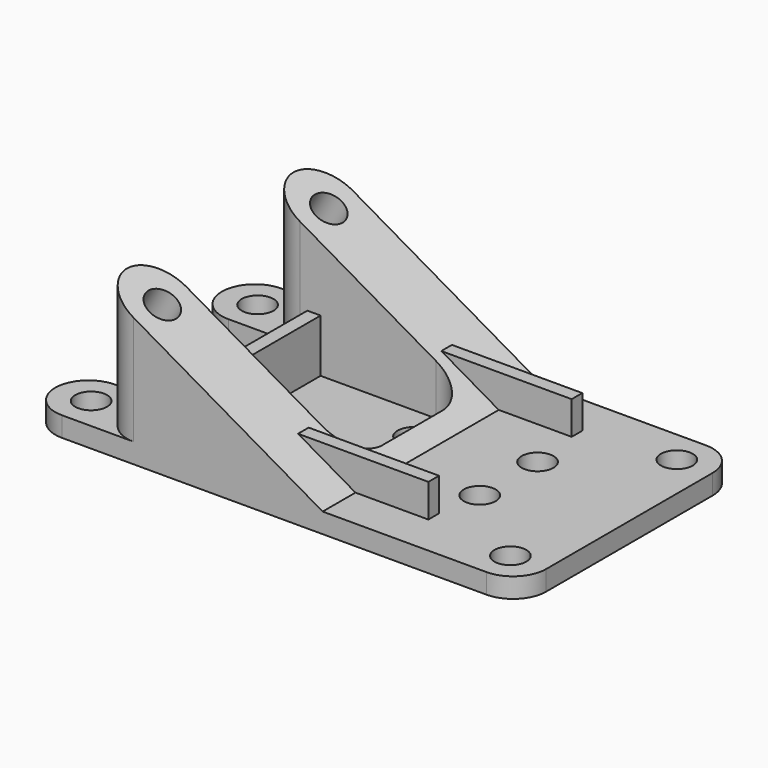
from build123d import *

# Parameters (mm, degrees)
F0_W        = 3
F0_H        = 5
F1_DEPTH    = 25
F0_R        = 2.4
F2_DEPTH    = 3
F3_T4_DEPTH = 238.5325445422
F4_R        = 4.99999
F5_R        = 4.99999
F6_R        = 5
F8_DEPTH    = 5
F9_ANGLE    = -30
F10_ANGLE   = -30
F7_W        = 36.4
F7_H        = 25
F7_R        = 4.4
F7_R_2      = 2.4
F13_DEPTH   = 2
F14_DEPTH   = 8


# Not quite as in the source:
# - a fillet or chamfer that OpenCascade refuses, or shapes differently, is made with other operations: its cross-section is extruded or revolved along the edge and cut away or added
# - a fillet or chamfer is up to 0.001 mm smaller than in the source, because OpenCascade refuses the exact size


with BuildPart() as f1:
    # F0 (on Top) → F1 (new body)
    with BuildSketch(Plane.XY):
        Polygon((-26.2931033156, 20.6850649182), (-26.2931033156, 15.6850649182), (-26.2931033156, 10.6850649182), (4.2068966844, 10.6850649182), (4.2068966844, 15.6850649182), (4.2068966844, 20.6850649182), align=None)
        with BuildLine():
            ThreePointArc((-18.8931033156, 15.6850649182), (-21.2931033156, 13.2850649182), (-23.6931033156, 15.6850649182))
            ThreePointArc((-23.6931033156, 15.6850649182), (-21.2931033156, 18.0850649182), (-18.8931033156, 15.6850649182))
        make_face(mode=Mode.SUBTRACT)
        Polygon((4.2068966844, -20.6850649182), (4.2068966844, -10.6850649182), (-26.2931033156, -10.6850649182), (-26.2931033156, -15.6850649182), (-26.2931033156, -20.6850649182), align=None)
        with BuildLine():
            ThreePointArc((-18.8931033156, -15.6850649182), (-21.2931033156, -18.0850649182), (-23.6931033156, -15.6850649182))
            ThreePointArc((-23.6931033156, -15.6850649182), (-21.2931033156, -13.2850649182), (-18.8931033156, -15.6850649182))
        make_face(mode=Mode.SUBTRACT)
        Polygon((4.2068966844, 15.6850649182), (4.2068966844, 10.6850649182), (4.2068966844, -10.6850649182), (4.2068966844, -20.6850649182), (7.2068966844, -20.6850649182), (7.2068966844, 15.6850649182), align=None)
        with BuildLine():
            ThreePointArc((-18.8931033156, 15.6850649182), (-21.2931033156, 18.0850649182), (-23.6931033156, 15.6850649182))
            ThreePointArc((-23.6931033156, 15.6850649182), (-21.2931033156, 13.2850649182), (-18.8931033156, 15.6850649182))
        make_face()
        with BuildLine():
            ThreePointArc((-18.8931033156, -15.6850649182), (-21.2931033156, -13.2850649182), (-23.6931033156, -15.6850649182))
            ThreePointArc((-23.6931033156, -15.6850649182), (-21.2931033156, -18.0850649182), (-18.8931033156, -15.6850649182))
        make_face()
        with Locations((5.7068966844, 18.1850649182)):
            Rectangle(F0_W, F0_H)
    extrude(amount=F1_DEPTH)

    # F0 (on Top) → F2 (join)
    with BuildSketch(Plane.XY):
        Polygon((-26.2931033156, 10.6850649182), (-26.2931033156, 15.6850649182), (-26.2931033156, 20.6850649182), (-37.0931033156, 20.6850649182), (-37.0931033156, 10.6850649182), align=None)
        with Locations((-31.6931033156, 15.6850649182)):
            Circle(F0_R, mode=Mode.SUBTRACT)
        Polygon((-26.2931033156, -15.6850649182), (-26.2931033156, -10.6850649182), (-37.0931033156, -10.6850649182), (-37.0931033156, -20.6850649182), (-26.2931033156, -20.6850649182), align=None)
        with Locations((-31.6931033156, -15.6850649182)):
            Circle(F0_R, mode=Mode.SUBTRACT)
        Polygon((36.9068966844, 20.6850649182), (7.2068966844, 20.6850649182), (7.2068966844, 15.6850649182), (7.2068966844, -20.6850649182), (36.9068966844, -20.6850649182), align=None)
        with Locations((31.5068966844, -15.6850649182)):
            Circle(F0_R, mode=Mode.SUBTRACT)
        with Locations((19.0568966844, -5.9)):
            Circle(F0_R, mode=Mode.SUBTRACT)
        with Locations((19.0568966844, 5)):
            Circle(F0_R, mode=Mode.SUBTRACT)
        with BuildLine():
            ThreePointArc((29.1068966844, 15.6850649182), (31.5068966844, 18.0850649182), (33.9068966844, 15.6850649182))
            ThreePointArc((33.9068966844, 15.6850649182), (31.5068966844, 13.2850649182), (29.1068966844, 15.6850649182))
        make_face(mode=Mode.SUBTRACT)
    extrude(amount=F2_DEPTH)

    # F3: chamfer of 22 x 38.1051177665 on 1 edges, made by hand


with BuildPart() as f3_tool2:
    # F3_s3 → F3_t4 (new body)
    with BuildSketch(Plane.XZ.offset(119.2662722711)):
        Polygon((7.2068966844, 3), (-30.8982210821, 25), (7.2068966844, 25), align=None)
    extrude(amount=-F3_T4_DEPTH)

    split(bisect_by=Plane.XY.offset(3), keep=Keep.TOP)


with BuildPart() as f1_1:
    add(f1.part)

    # F3_t1: cut F3_tool2
    add(f3_tool2.part, mode=Mode.SUBTRACT)

    # F4 (radius 5 in the source; OpenCascade refuses exactly that, so slightly less here)
    f4_edges = [f1_1.edges().sort_by_distance(p)[0] for p in [
        (-37.093103, 20.685065, 1.5),
        (-37.093103, 10.685065, 1.5),
        (-37.093103, -10.685065, 1.5),
        (-37.093103, -20.685065, 1.5),
        (36.906897, -20.685065, 1.5),
        (36.906897, 20.685065, 1.5),
    ]]
    fillet(f4_edges, radius=F4_R)

    # F5 (radius 5 in the source; OpenCascade refuses exactly that, so slightly less here)
    f5_edges = [f1_1.edges().sort_by_distance(p)[0] for p in [
        (-26.293103, 20.685065, 12.670617),
        (-26.293103, 10.685065, 12.670617),
        (-26.293103, -10.685065, 12.670617),
        (-26.293103, -20.685065, 12.670617),
    ]]
    fillet(f5_edges, radius=F5_R)

    # F6
    f6_edges = [f1_1.edges().sort_by_distance(p)[0] for p in [
        (4.206897, 10.685065, 2.366025),
        (4.206897, -10.685065, 2.366025),
    ]]
    fillet(f6_edges, radius=F6_R)


with BuildPart() as f8:
    # F0 (on Top) → F8 (new body, symmetric)
    with BuildSketch(Plane.XY):
        with BuildLine():
            ThreePointArc((-18.8931033156, 15.6850649182), (-21.2931033156, 18.0850649182), (-23.6931033156, 15.6850649182))
            ThreePointArc((-23.6931033156, 15.6850649182), (-21.2931033156, 13.2850649182), (-18.8931033156, 15.6850649182))
        make_face()
    extrude(amount=F8_DEPTH, both=True)


with BuildPart() as f8b:
    # F0 (on Top) → F8, piece 2 (new body, symmetric)
    with BuildSketch(Plane.XY):
        with BuildLine():
            ThreePointArc((-18.8931033156, -15.6850649182), (-21.2931033156, -13.2850649182), (-23.6931033156, -15.6850649182))
            ThreePointArc((-23.6931033156, -15.6850649182), (-21.2931033156, -18.0850649182), (-18.8931033156, -15.6850649182))
        make_face()
    extrude(amount=F8_DEPTH, both=True)


with BuildPart() as f8b_1:
    # F9: moved
    add(f8b.part.rotate(Axis((-21.2931033156, -15.6850649182, 0), (0, -1, 0)), F9_ANGLE))


with BuildPart() as f8_1:
    # F10: moved
    add(f8.part.rotate(Axis((-21.2931033156, 15.6850649182, 0), (0, -1, 0)), F10_ANGLE))


with BuildPart() as f8b_2:
    # F11: moved
    add(f8b_1.part.moved(Location((0, 0, 18.7))))


with BuildPart() as f8_2:
    # F11: moved
    add(f8_1.part.moved(Location((0, 0, 18.7))))


with BuildPart() as f1_2:
    add(f1_1.part)

    # F12: cut F8, F8b
    add(f8_2.part, mode=Mode.SUBTRACT)
    add(f8b_2.part, mode=Mode.SUBTRACT)


with BuildPart() as f13:
    # F7 (on Top) → F13 (new body)
    with BuildSketch(Plane.XY):
        Polygon((18.2, -14.5), (18.2, -12.5), (-18.2, -12.5), (-18.2, 12.5), (18.2, 12.5), (18.2, 14.5), (-20.2, 14.5), (-20.2, -14.5), align=None)
        Rectangle(F7_W, F7_H)
        with Locations((0, -5.45)):
            Circle(F7_R, mode=Mode.SUBTRACT)
        with Locations((0, 5.45)):
            Circle(F7_R, mode=Mode.SUBTRACT)
        with Locations((0, 5.45)):
            Circle(F7_R)
        with Locations((0, 5.45)):
            Circle(F7_R_2, mode=Mode.SUBTRACT)
        with Locations((0, -5.45)):
            Circle(F7_R)
        with Locations((0, -5.45)):
            Circle(F7_R_2, mode=Mode.SUBTRACT)
    extrude(amount=-F13_DEPTH)

    # F7 (on Top) → F14 (join)
    with BuildSketch(Plane.XY):
        Polygon((18.2, -14.5), (18.2, -12.5), (-18.2, -12.5), (-18.2, 12.5), (18.2, 12.5), (18.2, 14.5), (-20.2, 14.5), (-20.2, -14.5), align=None)
    extrude(amount=F14_DEPTH)


solid = Compound([f1_2.part, f13.part])
